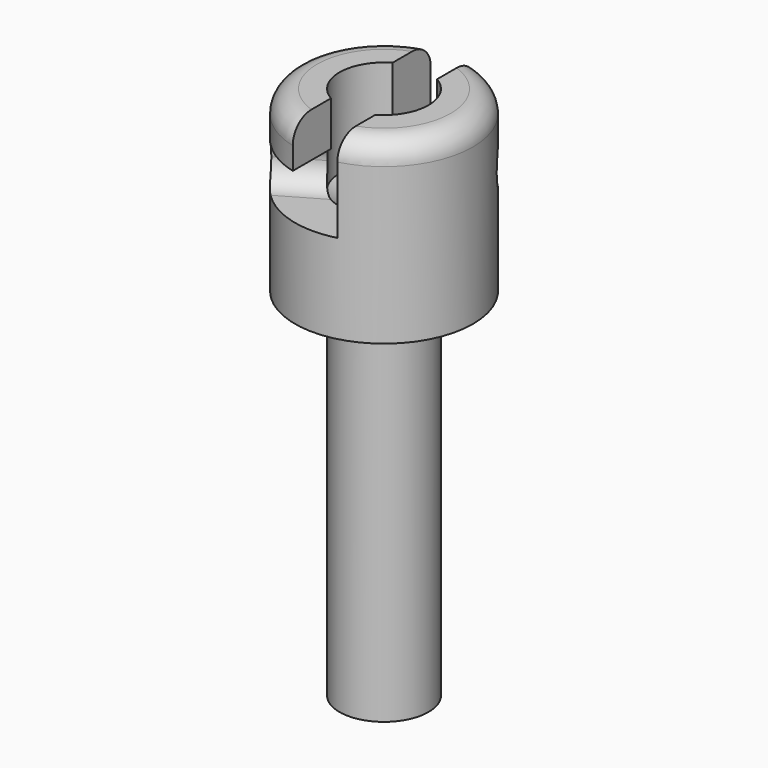
from build123d import *

# Parameters (mm, degrees)
F0_R          = 6.35
F1_DEPTH      = 12.7
F2_R          = 3.175
F3_DEPTH      = 25.4
F5_D          = 6.35
F5_DEPTH      = 6.35
F5_TIP        = 1.9077324654
F7_DEPTH      = 6.35
F10_W         = 4.7625
F10_H         = 3.175
F10_W_2       = 4.7752
F11_ANGLE     = 60
F12_T4_DEPTH  = 11.1125
F12_S5_R      = 6.35
F12_T6_DEPTH  = 8
F12_S7_R      = 3.175
F12_T8_DEPTH  = 8
F12_T12_DEPTH = 11.1125
F12_S13_R     = 6.35
F12_T14_DEPTH = 8
F12_S15_R     = 3.175
F12_T16_DEPTH = 8
F12_T20_DEPTH = 11.1125
F12_S21_R     = 6.35
F12_T22_DEPTH = 8
F12_S23_R     = 3.175
F12_T24_DEPTH = 8
F12_T28_DEPTH = 11.1125
F12_S29_R     = 6.35
F12_T30_DEPTH = 8
F12_S31_R     = 3.175
F12_T32_DEPTH = 8
F13_R         = 1.5875


# Not quite as in the source:
# - a fillet or chamfer that OpenCascade refuses, or shapes differently, is made with other operations: its cross-section is extruded or revolved along the edge and cut away or added
# - a feature names something its author has since deleted; it is built from what else it names


with BuildPart() as f1:
    # F0 (on Top) → F1 (new body)
    with BuildSketch(Plane.XY):
        Circle(F0_R)
    extrude(amount=F1_DEPTH)

    # F5
    with Locations(Plane.XY.offset(12.7)):
        with Locations((0, 0)):
            Hole(F5_D / 2, depth=F5_DEPTH)
            with Locations((0, 0, -(F5_DEPTH + F5_TIP / 2))):  # 118° drill point
                Cone(0, F5_D / 2, F5_TIP, mode=Mode.SUBTRACT)

    # F6 (on face) → F7 (cut)
    with BuildSketch(Plane.XY.offset(12.7)):
        with BuildLine():
            Line((-1.5875, -2.749630657), (-1.5875, -6.1483610621))
            ThreePointArc((-1.5875, -6.1483610621), (-0.8001272573, -6.2993885713), (0, -6.35))
            ThreePointArc((0, -6.35), (0.8001272573, -6.2993885713), (1.5875, -6.1483610621))
            Line((1.5875, -6.1483610621), (1.5875, -2.749630657))
            ThreePointArc((1.5875, -2.749630657), (0, -3.175), (-1.5875, -2.749630657))
        make_face()
        with BuildLine():
            ThreePointArc((1.5875, 6.1483610621), (0.8001272573, 6.2993885713), (0, 6.35))
            ThreePointArc((0, 6.35), (-0.8001272573, 6.2993885713), (-1.5875, 6.1483610621))
            Line((-1.5875, 6.1483610621), (-1.5875, 2.749630657))
            ThreePointArc((-1.5875, 2.749630657), (0, 3.175), (1.5875, 2.749630657))
            Line((1.5875, 2.749630657), (1.5875, 6.1483610621))
        make_face()
    extrude(amount=-F7_DEPTH, mode=Mode.SUBTRACT)

    # F10 (on face) → F11 (revolve, cut)
    with BuildSketch(Plane.YZ):
        with Locations((-3.96875, 7.9375)):
            Rectangle(F10_W, F10_H)
        with Locations((3.9624, 7.9375)):
            Rectangle(F10_W_2, F10_H)
    revolve(axis=Axis((0, 0, 6.35), (0, 0, -1)), revolution_arc=F11_ANGLE, mode=Mode.SUBTRACT)

    # F12: fillet of radius 1.5875 on 4 edges, made by hand


with BuildPart() as f3:
    # F2 (on Top) → F3 (new body)
    with BuildSketch(Plane.XY):
        Circle(F2_R)
    extrude(amount=-F3_DEPTH)


with BuildPart() as f12_tool2:
    # F12_s3 → F12_t4 (new body)
    with BuildSketch(Plane(origin=(0.6874076643, 0.396875, 0), x_dir=(0, 0, 1), z_dir=(-0.8660254038, -0.5, 0))):
        with BuildLine():
            ThreePointArc((7.9375, 0), (9.0600320151, -0.4649679849), (9.525, -1.5875))
            Line((9.525, -1.5875), (9.525, 0))
            Line((9.525, 0), (7.9375, 0))
        make_face()
    extrude(amount=F12_T4_DEPTH)

    # F12_s5 → F12_t6 (intersect, symmetric)
    with BuildSketch(Plane.XY.offset(8.7)):
        Circle(F12_S5_R)
    extrude(amount=F12_T6_DEPTH, both=True, mode=Mode.INTERSECT)

    # F12_s7 → F12_t8 (cut, symmetric)
    with BuildSketch(Plane.XY.offset(8.7)):
        Circle(F12_S7_R)
    extrude(amount=F12_T8_DEPTH, both=True, mode=Mode.SUBTRACT)


with BuildPart() as f1_1:
    add(f1.part)

    # F12_t1: union F12_tool2
    add(f12_tool2.part)


with BuildPart() as f12_tool10:
    # F12_s11 → F12_t12 (new body)
    with BuildSketch(Plane(origin=(-8.9362996353, -5.159375, 0), x_dir=(0, 0, 1), z_dir=(0.8660254038, 0.5, 0))):
        with BuildLine():
            ThreePointArc((6.35, 1.5875), (6.8149679849, 0.4649679849), (7.9375, 0))
            Line((7.9375, 0), (6.35, 0))
            Line((6.35, 0), (6.35, 1.5875))
        make_face()
    extrude(amount=F12_T12_DEPTH)

    # F12_s13 → F12_t14 (intersect, symmetric)
    with BuildSketch(Plane.XY.offset(7.1)):
        Circle(F12_S13_R)
    extrude(amount=F12_T14_DEPTH, both=True, mode=Mode.INTERSECT)

    # F12_s15 → F12_t16 (cut, symmetric)
    with BuildSketch(Plane.XY.offset(7.1)):
        Circle(F12_S15_R)
    extrude(amount=F12_T16_DEPTH, both=True, mode=Mode.SUBTRACT)


with BuildPart() as f1_2:
    add(f1_1.part)

    # F12_t9: union F12_tool10
    add(f12_tool10.part)


with BuildPart() as f12_tool18:
    # F12_s19 → F12_t20 (new body)
    with BuildSketch(Plane(origin=(8.9362996353, 5.159375, 0), x_dir=(0, 0, 1), z_dir=(-0.8660254038, -0.5, 0))):
        with BuildLine():
            ThreePointArc((7.9375, 0), (9.0600320151, 0.4649679849), (9.525, 1.5875))
            Line((9.525, 1.5875), (9.525, 0))
            Line((9.525, 0), (7.9375, 0))
        make_face()
    extrude(amount=F12_T20_DEPTH)

    # F12_s21 → F12_t22 (intersect, symmetric)
    with BuildSketch(Plane.XY.offset(8.7)):
        Circle(F12_S21_R)
    extrude(amount=F12_T22_DEPTH, both=True, mode=Mode.INTERSECT)

    # F12_s23 → F12_t24 (cut, symmetric)
    with BuildSketch(Plane.XY.offset(8.7)):
        Circle(F12_S23_R)
    extrude(amount=F12_T24_DEPTH, both=True, mode=Mode.SUBTRACT)


with BuildPart() as f1_3:
    add(f1_2.part)

    # F12_t17: union F12_tool18
    add(f12_tool18.part)


with BuildPart() as f12_tool26:
    # F12_s27 → F12_t28 (new body)
    with BuildSketch(Plane(origin=(-0.6874076643, -0.396875, 0), x_dir=(0, 0, 1), z_dir=(0.8660254038, 0.5, 0))):
        with BuildLine():
            ThreePointArc((6.35, -1.5875), (6.8149679849, -0.4649679849), (7.9375, 0))
            Line((7.9375, 0), (6.35, 0))
            Line((6.35, 0), (6.35, -1.5875))
        make_face()
    extrude(amount=F12_T28_DEPTH)

    # F12_s29 → F12_t30 (intersect, symmetric)
    with BuildSketch(Plane.XY.offset(7.1)):
        Circle(F12_S29_R)
    extrude(amount=F12_T30_DEPTH, both=True, mode=Mode.INTERSECT)

    # F12_s31 → F12_t32 (cut, symmetric)
    with BuildSketch(Plane.XY.offset(7.1)):
        Circle(F12_S31_R)
    extrude(amount=F12_T32_DEPTH, both=True, mode=Mode.SUBTRACT)


with BuildPart() as f1_4:
    add(f1_3.part)

    # F12_t25: union F12_tool26
    add(f12_tool26.part)

    # F13
    f13_edges = [f1_4.edges().sort_by_distance(p)[0] for p in [
        (-6.35, 0, 12.7),
        (5.020116, 3.888565, 12.7),
        (5.020116, -3.888565, 12.7),
    ]]
    fillet(f13_edges, radius=F13_R)


solid = Compound([f3.part, f1_4.part])
